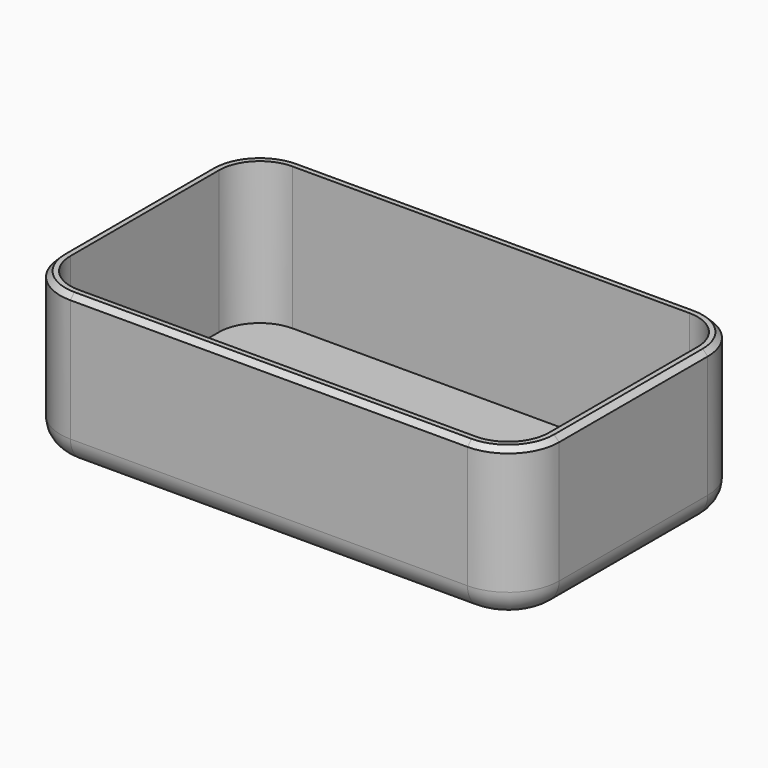
from build123d import *

# Parameters (mm, degrees)
F1_DEPTH = 30
F2_T     = -2
F3_R     = 5
F4_SIZE  = 1
F6_DEPTH = 0.4


# Not quite as in the source:
# - ends of sketch curves that miss each other by under 0.0002 mm in the source are joined


with BuildPart() as f1:
    # F0 (on Top) → F1 (new body)
    with BuildSketch(Plane.XY):
        with BuildLine():
            Line((38.72, 30.375), (-39.28, 30.375))
            ThreePointArc((-39.28, 30.375), (-46.3510678119, 27.4460678119), (-49.28, 20.375))
            Line((-49.28, 20.375), (-49.28, -16.125))
            ThreePointArc((-49.28, -16.125), (-46.3510678119, -23.1960678119), (-39.28, -26.125))
            Line((-39.28, -26.125), (38.72, -26.125))
            ThreePointArc((38.72, -26.125), (45.7910678119, -23.1960678119), (48.72, -16.125))
            Line((48.72, -16.125), (48.72, 20.375))
            ThreePointArc((48.72, 20.375), (45.7910678119, 27.4460678119), (38.72, 30.375))
        make_face()
    extrude(amount=F1_DEPTH)

    # F2
    f2_openings = [f1.faces().sort_by_distance(p)[0] for p in [
        (-0.28, 2.125, 30),
    ]]
    offset(amount=F2_T, openings=f2_openings)

    # F3
    f3_edges = [f1.edges().sort_by_distance(p)[0] for p in [
        (-0.28, -26.125, 0),
    ]]
    fillet(f3_edges, radius=F3_R)

    # F4
    f4_edges = [f1.edges().sort_by_distance(p)[0] for p in [
        (-0.28, -26.125, 30),
        (-46.351068, -23.196068, 30),
        (-49.28, 2.125, 30),
        (-46.351068, 27.446068, 30),
        (-0.28, 30.375, 30),
        (45.791068, 27.446068, 30),
        (48.72, 2.125, 30),
        (45.791068, -23.196068, 30),
    ]]
    chamfer(f4_edges, length=F4_SIZE)

    # F5 (on face) → F6 (cut)
    with BuildSketch(Plane(origin=(0, 0, 0), x_dir=(1, 0, 0), z_dir=(0, 0, -1))):
        with BuildLine():
            add(Edge.make_bspline(
                [(-8.093493, 9.19317), (-4.0467455, 12.8119), (2e-06, 12.8119), (4.0467495, 12.8119), (8.093497, 9.19317)],
                knots=[0, 0, 0, 0, 0.5, 1, 1, 1, 1], degree=3))
            Line((-8.093493, 9.19317), (0, 1.099674))
            Line((0, 1.099674), (8.093497, 9.19317))
        make_face()
        Polygon((-1.313547, 1e-06), (-9.40704, 8.093494), (-17.499982, 1e-06), (-9.40704, -8.092941), align=None)
        Polygon((17.499982, 1e-06), (9.406489, 8.093494), (1.312996, 1e-06), (9.406489, -8.092941), align=None)
        with BuildLine():
            Line((8.093495, -9.193168), (0, -1.099672))
            Line((0, -1.099672), (-8.093493, -9.193168))
            add(Edge.make_bspline(
                [(-8.093493, -9.193168), (-4.0467455, -12.811898), (2e-06, -12.811898), (4.0467495, -12.811898), (8.093495, -9.193168)],
                knots=[0, 0, 0, 0, 0.5, 1, 1, 1, 1], degree=3))
        make_face()
    extrude(amount=-F6_DEPTH, mode=Mode.SUBTRACT)


solid = f1.part
